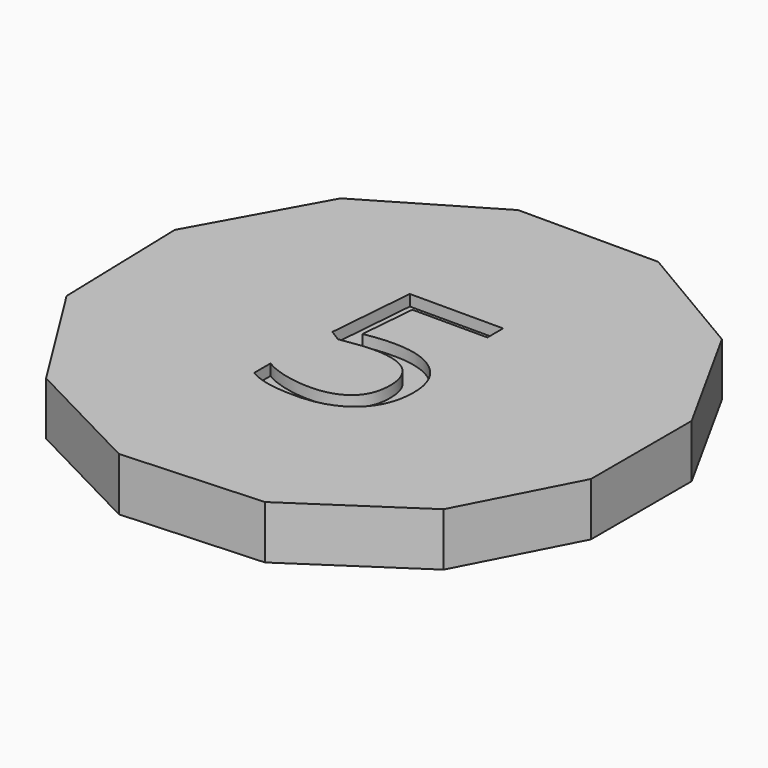
from build123d import *

# Parameters (mm, degrees)
F1_DEPTH     = 2.4
F2_TEXT_SIZE = 11.8598565642
F3_DEPTH     = 0.5


# Not quite as in the source:
# - Text() gives the source's letters only with a copy of the font that has no kerning and outlines rounded to 1/6400 em; it was checked with that copy


with BuildPart() as f1:
    # F0 (on Top) → F1 (new body)
    with BuildSketch(Plane.XY):
        Polygon((3.1589271694, 11.5767516661), (-3.1589271694, 11.5767516661), (-8.6011601655, 8.3677980262), (-11.6592421479, 2.8393789), (-11.4855049976, -3.4760861541), (-8.128106823, -8.8280167351), (-2.5176830392, -11.7329140504), (3.7906159678, -11.3855711576), (9.0481961498, -7.8822678484), (11.6592421479, -2.8393789), (11.6592421479, 2.8393789), (8.6011601655, 8.3677980262), align=None)
    extrude(amount=F1_DEPTH)

    # F2 (on face) → F3 (cut)
    with BuildSketch(Plane.XY.offset(2.4)):
        with Locations((-3.4337990959, -4.2695483631)):
            Text('5', F2_TEXT_SIZE, font='Open Sans', text_align=(TextAlign.LEFT, TextAlign.BOTTOM))
    extrude(amount=-F3_DEPTH, mode=Mode.SUBTRACT)


solid = f1.part
